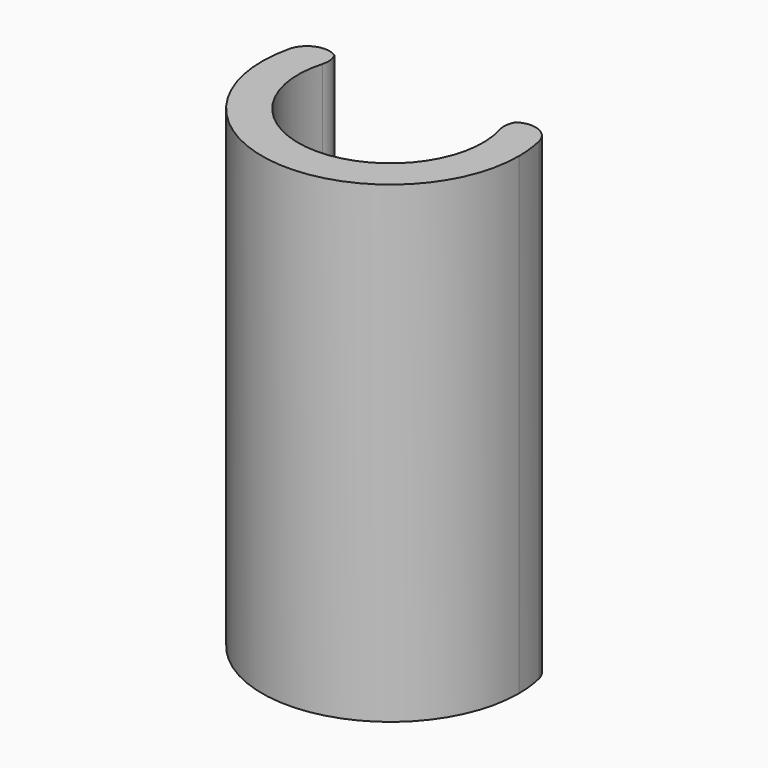
from build123d import *

# Parameters (mm, degrees)
F1_DEPTH    = 21
F2_T1_DEPTH = 23.8690975764
F2_T3_DEPTH = 30.409576176


# Not quite as in the source:
# - a fillet or chamfer that OpenCascade refuses, or shapes differently, is made with other operations: its cross-section is extruded or revolved along the edge and cut away or added


with BuildPart() as f1:
    # F0 (on Top) → F1 (new body)
    with BuildSketch(Plane.XY):
        with BuildLine():
            ThreePointArc((3.7440062904, 1.6710526316), (4.0100140767, 0.8542757779), (4.1, 0))
            ThreePointArc((4.1, 0), (-0.8542757779, -4.0100140767), (-3.7440062904, 1.6710526316))
            ThreePointArc((-3.7440062904, 1.6710526316), (-4.335673559, 2.3159292575), (-4.8175607103, 3.0464912281))
            ThreePointArc((-4.8175607103, 3.0464912281), (-1.5858600114, -5.4749473079), (5.7, 0))
            ThreePointArc((5.7, 0), (5.4749473079, 1.5858600114), (4.8175607103, 3.0464912281))
            ThreePointArc((4.8175607103, 3.0464912281), (4.335673559, 2.3159292575), (3.7440062904, 1.6710526316))
        make_face()
    extrude(amount=F1_DEPTH)

    # F2: fillet of radius 1 on 4 edges, made by hand

    # F2_s2 → F2_t1 (cut)
    with BuildSketch(Plane.XY.offset(-1.4345487882)):
        with BuildLine():
            ThreePointArc((-4.1434007569, 2.0830634278), (-3.9202406694, 1.6409302608), (-3.9366000062, 1.1459408325))
            ThreePointArc((-3.9366000062, 1.1459408325), (-3.8492679656, 1.4117847318), (-3.7440062904, 1.6710526316))
            ThreePointArc((-3.7440062904, 1.6710526316), (-3.9490803621, 1.8718458373), (-4.1434007569, 2.0830634278))
        make_face()
        with BuildLine():
            ThreePointArc((4.1434007569, 2.0830634278), (3.9202406694, 1.6409302608), (3.9366000062, 1.1459408325))
            ThreePointArc((3.9366000062, 1.1459408325), (3.8492679656, 1.4117847318), (3.7440062904, 1.6710526316))
            ThreePointArc((3.7440062904, 1.6710526316), (3.9490803621, 1.8718458373), (4.1434007569, 2.0830634278))
        make_face()
    extrude(amount=F2_T1_DEPTH, mode=Mode.SUBTRACT)

    # F2_s4 → F2_t3 (cut)
    with BuildSketch(Plane.XY.offset(-4.704788088)):
        with BuildLine():
            ThreePointArc((-5.5470205992, 1.3117021277), (-4.849273554, 2.0429045287), (-3.8701884613, 1.7921052632))
            ThreePointArc((-3.8701884613, 1.7921052632), (-4.3889198505, 2.3852779082), (-4.8175607103, 3.0464912281))
            ThreePointArc((-4.8175607103, 3.0464912281), (-5.2543800525, 2.2094094831), (-5.5470205992, 1.3117021277))
        make_face()
        with BuildLine():
            ThreePointArc((3.8701884613, 1.7921052632), (4.849273554, 2.0429045287), (5.5470205992, 1.3117021277))
            ThreePointArc((5.5470205992, 1.3117021277), (5.2543800525, 2.2094094831), (4.8175607103, 3.0464912281))
            ThreePointArc((4.8175607103, 3.0464912281), (4.3889198505, 2.3852779082), (3.8701884613, 1.7921052632))
        make_face()
    extrude(amount=F2_T3_DEPTH, mode=Mode.SUBTRACT)


solid = f1.part
